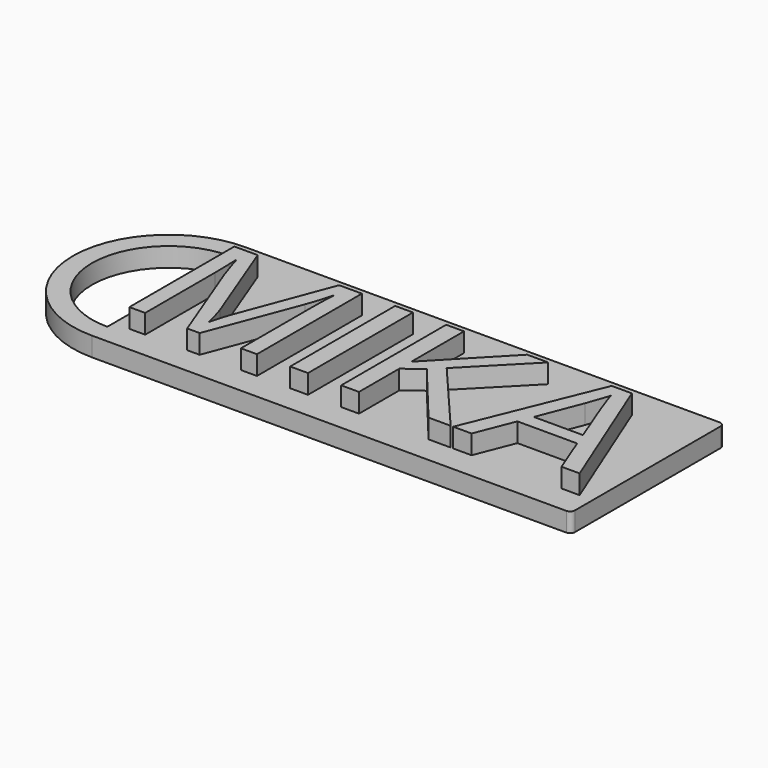
from build123d import *

# Parameters (mm, degrees)
F4_DEPTH     = 2
F1_R         = 0.5
F2_TEXT_SIZE = 19.9029730066
F3_DEPTH     = 2


# Not quite as in the source:
# - Text() gives the source's letters only with a copy of the font that has no kerning and outlines rounded to 1/6400 em; it was checked with that copy


with BuildPart() as f4:
    # F0 (on Top) → F4 (new body)
    with BuildSketch(Plane.XY):
        Polygon((44.7291392038, 3.2207785361), (-5.2708607962, 3.2207785361), (-5.2708607962, 1.2207785361), (-5.2708607962, -14.7792214639), (-5.2708607962, -16.7792214639), (44.7291392038, -16.7792214639), align=None)
        with BuildLine():
            Line((-5.2708607962, 1.2207785361), (-5.2708607962, 3.2207785361))
            ThreePointArc((-5.2708607962, 3.2207785361), (-15.2708607962, -6.7792214639), (-5.2708607962, -16.7792214639))
            Line((-5.2708607962, -16.7792214639), (-5.2708607962, -14.7792214639))
            ThreePointArc((-5.2708607962, -14.7792214639), (-13.2708607962, -6.7792214639), (-5.2708607962, 1.2207785361))
        make_face()
    extrude(amount=F4_DEPTH)

    # F1
    f1_edges = [f4.edges().sort_by_distance(p)[0] for p in [
        (44.729139, -16.779221, 1),
        (44.729139, 3.220779, 1),
    ]]
    fillet(f1_edges, radius=F1_R)

    # F2 (on face) → F3 (join)
    with BuildSketch(Plane.XY.offset(2)):
        with Locations((-5.2708607962, -13.9442917463)):
            Text('MIKA', F2_TEXT_SIZE, font='Arimo', text_align=(TextAlign.LEFT, TextAlign.BOTTOM))
    extrude(amount=F3_DEPTH)


solid = f4.part
